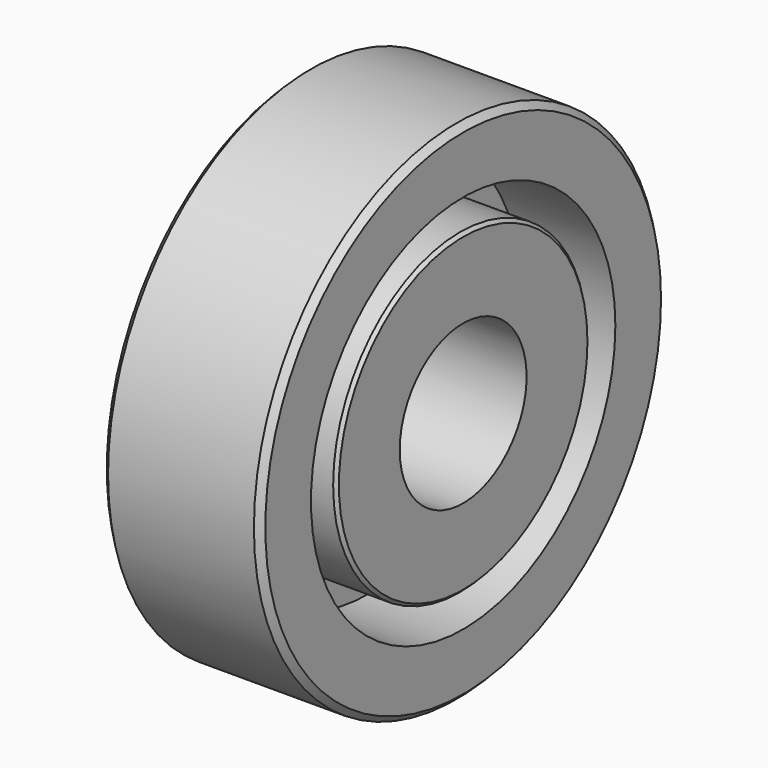
from build123d import *

# Parameters (mm, degrees)
F0_R     = 40
F1_DEPTH = 25
F2_R     = 12.5
F3_DEPTH = 25.001
F4_SIZE  = 1
F5_R     = 30
F5_R_2   = 25
F6_DEPTH = 15
F8_SIZE  = 0.5
F9_DEPTH = 10


# Not quite as in the source:
# - two fillets or chamfers of one size are made in one step


with BuildPart() as f1:
    # F0 (on Right) → F1 (new body)
    with BuildSketch(Plane.YZ):
        Circle(F0_R)
    extrude(amount=F1_DEPTH)

    # F2 (on face) → F3 (cut, through all)
    with BuildSketch(Plane(origin=(0, 0, 0), x_dir=(0, -1, 0), z_dir=(-1, 0, 0))):
        Circle(F2_R)
    extrude(amount=-F3_DEPTH, mode=Mode.SUBTRACT)

    # F4
    f4_edges = [f1.edges().sort_by_distance(p)[0] for p in [
        (0, -40, 0),
        (25, -40, 0),
    ]]
    chamfer(f4_edges, length=F4_SIZE)

    # F5 (on face) → F6 (cut)
    with BuildSketch(Plane.YZ.offset(25)):
        Circle(F5_R)
        Circle(F5_R_2, mode=Mode.SUBTRACT)
    extrude(amount=-F6_DEPTH, mode=Mode.SUBTRACT)

    # F8
    f8_edges = [f1.edges().sort_by_distance(p)[0] for p in [
        (25, -25, 0),
    ]]
    chamfer(f8_edges, length=F8_SIZE)

    # F5 (on face) → F9 (cut)
    with BuildSketch(Plane.YZ.offset(25)):
        Circle(F5_R)
        Circle(F5_R_2, mode=Mode.SUBTRACT)
    extrude(amount=-F9_DEPTH, mode=Mode.SUBTRACT)


solid = f1.part
